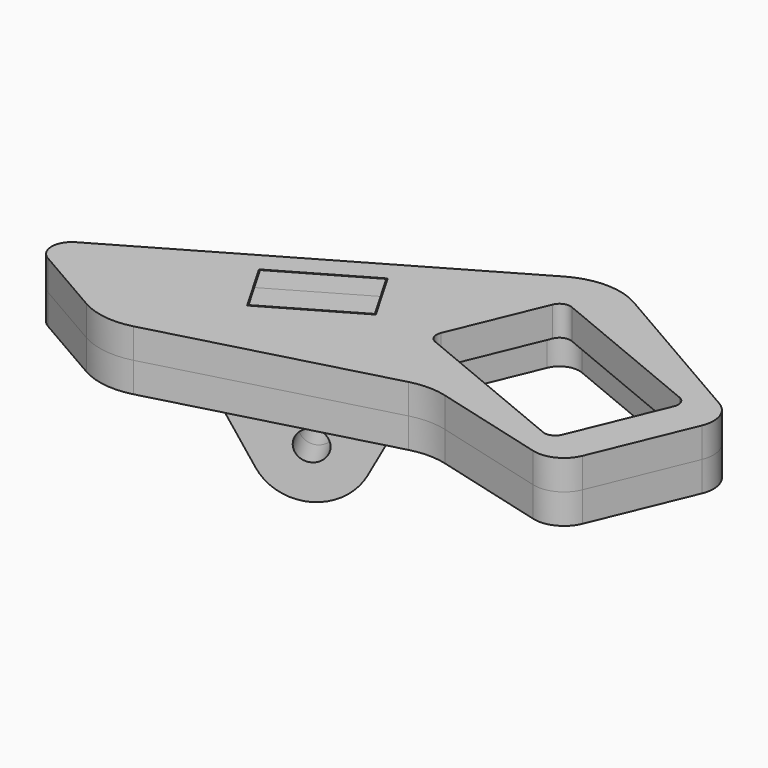
from build123d import *

# Parameters (mm, degrees)
F1_DEPTH  = 3
F3_DEPTH  = 3
F6_R      = 1.5
F6_W      = 10
F6_H      = 6
F7_DEPTH  = 3
F9_OFFSET = 0.1


with BuildPart() as f1:
    # F0 (on Top) → F1 (new body)
    with BuildSketch(Plane.XY):
        with BuildLine():
            Line((-3.5, 21.0732848254), (-37, 1.7320508076))
            ThreePointArc((-37, 1.7320508076), (-38, 0), (-37, -1.7320508076))
            Line((-37, -1.7320508076), (-29.8315443489, -5.8707606074))
            ThreePointArc((-29.8315443489, -5.8707606074), (-27.2452276945, -6.7486968105), (-24.5198110332, -6.5700635649))
            Line((-24.5198110332, -6.5700635649), (-1.8117333157, -0.4854524788))
            ThreePointArc((-1.8117333157, -0.4854524788), (0, -0.2469332629), (1.8117333157, -0.4854524788))
            Line((1.8117333157, -0.4854524788), (13.0880962857, -3.5069448302))
            ThreePointArc((13.0880962857, -3.5069448302), (15.1914194917, -3.299785576), (16.6361920186, -1.7572176484))
            Line((16.6361920186, -1.7572176484), (20.725816557, 8.1160093774))
            ThreePointArc((20.725816557, 8.1160093774), (20.794968348, 10.2283780704), (19.4541779595, 11.8621358858))
            Line((19.4541779595, 11.8621358858), (3.5, 21.0732848254))
            ThreePointArc((3.5, 21.0732848254), (0, 22.0111069989), (-3.5, 21.0732848254))
        make_face()
        with BuildLine():
            Line((17.8162192325, 8.9309978447), (13.9893849089, -0.3077974804))
            ThreePointArc((13.9893849089, -0.3077974804), (12.9069927086, -1.3901896807), (11.3762589791, -1.3901896807))
            Line((11.3762589791, -1.3901896807), (-4.7916328398, 5.3067703857))
            ThreePointArc((-4.7916328398, 5.3067703857), (-5.8740250401, 6.389162586), (-5.8740250401, 7.9198963155))
            Line((-5.8740250401, 7.9198963155), (-2.0471907165, 17.1586916406))
            ThreePointArc((-2.0471907165, 17.1586916406), (-0.9647985162, 18.2410838409), (0.5659352133, 18.2410838409))
            Line((0.5659352133, 18.2410838409), (16.7338270322, 11.5441237745))
            ThreePointArc((16.7338270322, 11.5441237745), (17.8162192325, 10.4617315742), (17.8162192325, 8.9309978447))
        make_face(mode=Mode.SUBTRACT)
    extrude(amount=F1_DEPTH)


with BuildPart() as f3:
    # F2 (on face) → F3 (new body)
    with BuildSketch(Plane.XY.offset(3)):
        with BuildLine():
            Line((1.8117333157, -0.4854524788), (13.0880962857, -3.5069448302))
            ThreePointArc((13.0880962857, -3.5069448302), (15.1914194917, -3.299785576), (16.6361920186, -1.7572176484))
            Line((16.6361920186, -1.7572176484), (20.725816557, 8.1160093774))
            ThreePointArc((20.725816557, 8.1160093774), (20.794968348, 10.2283780704), (19.4541779595, 11.8621358858))
            Line((19.4541779595, 11.8621358858), (3.5, 21.0732848254))
            ThreePointArc((3.5, 21.0732848254), (0, 22.0111069989), (-3.5, 21.0732848254))
            Line((-3.5, 21.0732848254), (-37, 1.7320508076))
            ThreePointArc((-37, 1.7320508076), (-38, 0), (-37, -1.7320508076))
            Line((-37, -1.7320508076), (-29.8315443489, -5.8707606074))
            ThreePointArc((-29.8315443489, -5.8707606074), (-27.2452276945, -6.7486968105), (-24.5198110332, -6.5700635649))
            Line((-24.5198110332, -6.5700635649), (-1.8117333157, -0.4854524788))
            ThreePointArc((-1.8117333157, -0.4854524788), (0, -0.2469332629), (1.8117333157, -0.4854524788))
        make_face()
        with BuildLine():
            ThreePointArc((-4.4472177507, 6.138261965), (-5.0425334609, 6.7335776751), (-5.0425334609, 7.5754812264))
            Line((-5.0425334609, 7.5754812264), (-1.2156991372, 16.8142765515))
            ThreePointArc((-1.2156991372, 16.8142765515), (-0.620383427, 17.4095922616), (0.2215201242, 17.4095922616))
            Line((0.2215201242, 17.4095922616), (16.3894119431, 10.7126321952))
            ThreePointArc((16.3894119431, 10.7126321952), (16.9847276533, 10.1173164851), (16.9847276533, 9.2754129339))
            Line((16.9847276533, 9.2754129339), (13.1578933296, 0.0366176088))
            ThreePointArc((13.1578933296, 0.0366176088), (12.5625776195, -0.5586981014), (11.7206740683, -0.5586981014))
            Line((11.7206740683, -0.5586981014), (-4.4472177507, 6.138261965))
        make_face(mode=Mode.SUBTRACT)
    extrude(amount=F3_DEPTH)


with BuildPart() as f7:
    # F6 (on offset) → F7 (new body)
    with BuildSketch(Plane(origin=(-8.75, 15.1554445662, 0), x_dir=(-0.8660254038, -0.5, 0), z_dir=(-0.5, 0.8660254038, 0))):
        with BuildLine():
            ThreePointArc((15.6119687021, -8.3087430662), (16.0336248853, -7.1884294616), (16.1769145362, -6))
            ThreePointArc((16.1769145362, -6), (9.9884850746, -1.1432896509), (6.7418603703, -8.3087430662))
            ThreePointArc((6.7418603703, -8.3087430662), (11.1769145362, -11), (15.6119687021, -8.3087430662))
        make_face()
        with Locations((11.1769145362, -6)):
            Circle(F6_R, mode=Mode.SUBTRACT)
        with BuildLine():
            ThreePointArc((6.7418603703, -8.3087430662), (9.9884850746, -1.1432896509), (16.1769145362, -6))
            ThreePointArc((16.1769145362, -6), (16.0336248853, -7.1884294616), (15.6119687021, -8.3087430662))
            Line((15.6119687021, -8.3087430662), (19.9372265739, 0))
            Line((19.9372265739, 0), (16.1769145362, 0))
            Line((16.1769145362, 0), (6.1769145362, 0))
            Line((6.1769145362, 0), (2.4166024986, 0))
            Line((2.4166024986, 0), (6.7418603703, -8.3087430662))
        make_face()
        with Locations((11.1769145362, 3)):
            Rectangle(F6_W, F6_H)
    extrude(amount=-F7_DEPTH)


with BuildPart() as f8_1:
    # F8: copy of F7
    add(f7.part.moved(Location((1.5, -2.5980762114, 0))))


with BuildPart() as f1_1:
    add(f1.part)

    # F9: cut F8_1, F7, each made larger all round first
    f9_tool = offset(f8_1.part, amount=F9_OFFSET, kind=Kind.INTERSECTION, mode=Mode.PRIVATE)
    add(f9_tool, mode=Mode.SUBTRACT)
    f9_tool1 = offset(f7.part, amount=F9_OFFSET, kind=Kind.INTERSECTION, mode=Mode.PRIVATE)
    add(f9_tool1, mode=Mode.SUBTRACT)


with BuildPart() as f3_1:
    add(f3.part)

    # F9: cut F8_1, F7, each made larger all round first
    f9_tool = offset(f8_1.part, amount=F9_OFFSET, kind=Kind.INTERSECTION, mode=Mode.PRIVATE)
    add(f9_tool, mode=Mode.SUBTRACT)
    f9_tool1 = offset(f7.part, amount=F9_OFFSET, kind=Kind.INTERSECTION, mode=Mode.PRIVATE)
    add(f9_tool1, mode=Mode.SUBTRACT)


solid = Compound([f7.part, f8_1.part, f1_1.part, f3_1.part])
